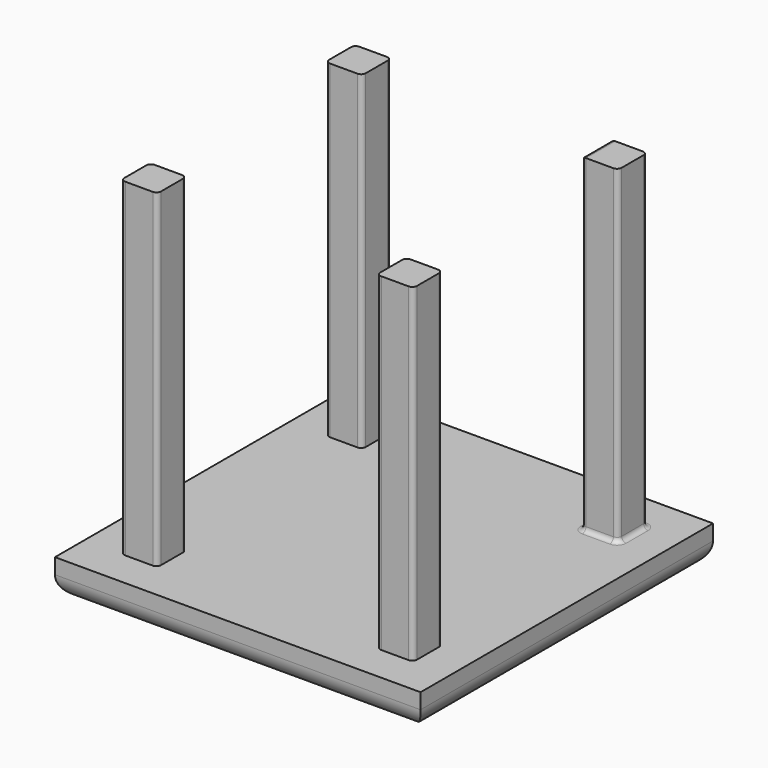
from build123d import *

# Parameters (mm, degrees)
F0_W     = 400
F0_H     = 400
F1_DEPTH = 40
F2_W     = 40
F2_H     = 40
F3_DEPTH = 360
F4_R     = 23.11
F5_R     = 5
F6_R     = 5


with BuildPart() as f1:
    # F0 (on Top) → F1 (new body)
    with BuildSketch(Plane.XY):
        with Locations((-9.5043759793, 29.5748232458)):
            Rectangle(F0_W, F0_H)
    extrude(amount=F1_DEPTH)

    # F2 (on face) → F3 (join)
    with BuildSketch(Plane.XY.offset(40)):
        with Locations((130.4956240207, -110.4251767542)):
            Rectangle(F2_W, F2_H)
        with Locations((-149.5043759793, -110.4251767542)):
            Rectangle(F2_W, F2_H)
        with Locations((-149.5043759793, 169.5748232458)):
            Rectangle(F2_W, F2_H)
        with Locations((130.4956240207, 169.5748232458)):
            Rectangle(F2_W, F2_H)
    extrude(amount=F3_DEPTH)

    # F4
    f4_edges = [f1.edges().sort_by_distance(p)[0] for p in [
        (-209.504376, 29.574823, 0),
        (-9.504376, 229.574823, 0),
        (-9.504376, -170.425177, 0),
        (190.495624, 29.574823, 0),
    ]]
    fillet(f4_edges, radius=F4_R)

    # F5
    f5_edges = [f1.edges().sort_by_distance(p)[0] for p in [
        (-129.504376, 189.574823, 220),
        (-129.504376, 149.574823, 220),
        (-169.504376, -130.425177, 220),
        (-129.504376, -130.425177, 220),
        (-129.504376, -90.425177, 220),
        (-169.504376, -90.425177, 220),
        (-169.504376, 189.574823, 220),
        (-169.504376, 149.574823, 220),
    ]]
    fillet(f5_edges, radius=F5_R)

    # F6
    f6_edges = [f1.edges().sort_by_distance(p)[0] for p in [
        (150.495624, -130.425177, 220),
        (150.495624, -90.425177, 220),
        (150.495624, 149.574823, 220),
        (150.495624, 189.574823, 220),
        (110.495624, 189.574823, 220),
        (110.495624, 149.574823, 220),
        (110.495624, 169.574823, 40),
        (110.495624, 169.574823, 400),
        (110.495624, -90.425177, 220),
        (110.495624, -130.425177, 220),
        (130.495624, 189.574823, 40),
        (130.495624, 149.574823, 40),
        (150.495624, 169.574823, 40),
    ]]
    fillet(f6_edges, radius=F6_R)


solid = f1.part
